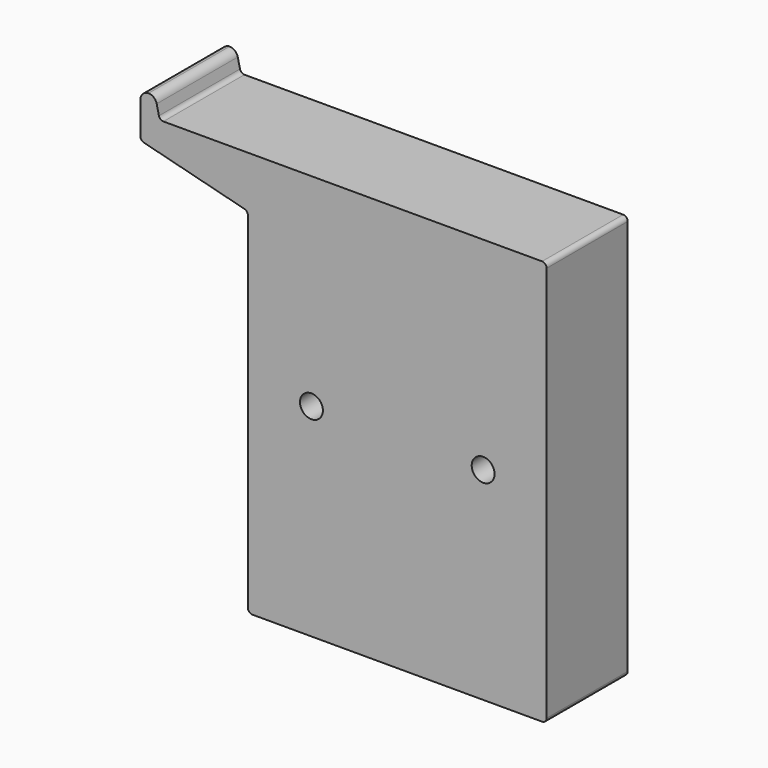
from build123d import *

# Parameters (mm, degrees)
F0_R        = 2
F1_DEPTH    = 17.7
F2_T1_DEPTH = 25.2
F2_T3_DEPTH = 23.679138459
F3_R        = 0.8


# Not quite as in the source:
# - a fillet or chamfer that OpenCascade refuses, or shapes differently, is made with other operations: its cross-section is extruded or revolved along the edge and cut away or added


with BuildPart() as f1:
    # F0 (on Front) → F1 (new body)
    with BuildSketch(Plane.XZ):
        Polygon((26.1, 35.4), (-41.5, 35.4), (-42.3, 38.9), (-44.9, 38.9), (-44.9, 31.2), (-26.1, 26.4), (-26.1, -35.4), (26.1, -35.4), align=None)
        with Locations((-15, 0)):
            Circle(F0_R, mode=Mode.SUBTRACT)
        with Locations((15, 0)):
            Circle(F0_R, mode=Mode.SUBTRACT)
    extrude(amount=-F1_DEPTH)

    # F2: fillet of radius 1.5 on 2 edges, made by hand

    # F2_s2 → F2_t1 (cut)
    with BuildSketch(Plane.XZ.offset(-21.45)):
        with BuildLine():
            ThreePointArc((-43.4, 38.9), (-44.4606601718, 38.4606601718), (-44.9, 37.4))
            Line((-44.9, 37.4), (-44.9, 38.9))
            Line((-44.9, 38.9), (-43.4, 38.9))
        make_face()
    extrude(amount=F2_T1_DEPTH, mode=Mode.SUBTRACT)

    # F2_s4 → F2_t3 (cut)
    with BuildSketch(Plane.XZ.offset(-20.6895692295)):
        with BuildLine():
            ThreePointArc((-42.0335399319, 37.7342372023), (-42.560775769, 38.5728929626), (-43.4958276918, 38.9))
            Line((-43.4958276918, 38.9), (-42.3, 38.9))
            Line((-42.3, 38.9), (-42.0335399319, 37.7342372023))
        make_face()
    extrude(amount=F2_T3_DEPTH, mode=Mode.SUBTRACT)

    # F3
    f3_edges = [f1.edges().sort_by_distance(p)[0] for p in [
        (-41.5, 8.85, 35.4),
        (26.1, 8.85, 35.4),
        (26.1, 8.85, -35.4),
        (-44.9, 8.85, 31.2),
        (-26.1, 8.85, 26.4),
        (-26.1, 8.85, -35.4),
    ]]
    fillet(f3_edges, radius=F3_R)


solid = f1.part
